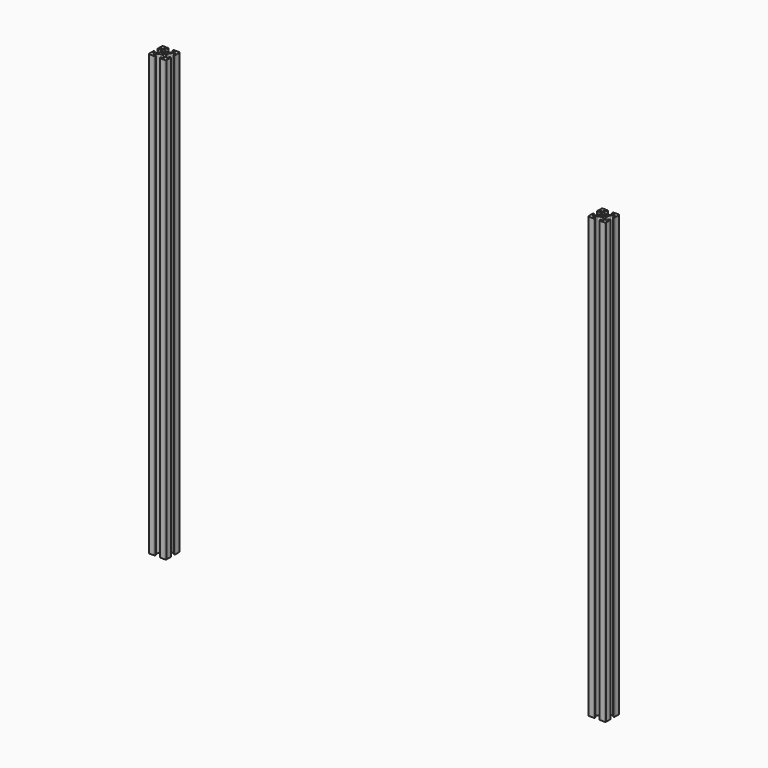
from build123d import *

# Parameters (mm, degrees)
F0_R     = 2.6035
F1_DEPTH = 635
F2_R     = 1.18109
F3_R     = 5.08
F4_R     = 0.762
F5_R     = 1.27


# Not quite as in the source:
# - a fillet or chamfer is up to 0.001 mm smaller than in the source, because OpenCascade refuses the exact size


with BuildPart() as f1:
    # F0 (on Top) → F1 (new body)
    with BuildSketch(Plane.XY):
        Polygon((12.7, 3.2385), (12.7, 12.7), (3.2385, 12.7), (3.2385, 10.3378), (8.7752354349, 10.3378), (2.9459354349, 4.5085), (-2.9459354349, 4.5085), (-8.7752354349, 10.3378), (-3.2385, 10.3378), (-3.2385, 12.7), (-12.7, 12.7), (-12.7, 3.2385), (-10.3378, 3.2385), (-10.3378, 8.7752354349), (-4.5085, 2.9459354349), (-4.5085, -2.9459354349), (-10.3378, -8.7752354349), (-10.3378, -3.2385), (-12.7, -3.2385), (-12.7, -12.7), (-3.2385, -12.7), (-3.2385, -10.3378), (-8.7752354349, -10.3378), (-2.9459354349, -4.5085), (2.9459354349, -4.5085), (8.7752354349, -10.3378), (3.2385, -10.3378), (3.2385, -12.7), (12.7, -12.7), (12.7, -3.2385), (10.3378, -3.2385), (10.3378, -8.7752354349), (4.5085, -2.9459354349), (4.5085, 2.9459354349), (10.3378, 8.7752354349), (10.3378, 3.2385), align=None)
        Circle(F0_R, mode=Mode.SUBTRACT)
    extrude(amount=F1_DEPTH)

    # F2 (radius 1.1811 in the source; OpenCascade refuses exactly that, so slightly less here)
    f2_edges = [f1.edges().sort_by_distance(p)[0] for p in [
        (3.2385, 12.7, 317.5),
        (3.2385, 10.3378, 317.5),
        (-3.2385, 12.7, 317.5),
        (-12.7, 3.2385, 317.5),
        (-3.2385, 10.3378, 317.5),
        (-10.3378, 3.2385, 317.5),
        (12.7, 3.2385, 317.5),
        (10.3378, 3.2385, 317.5),
        (12.7, -3.2385, 317.5),
        (10.3378, -3.2385, 317.5),
        (3.2385, -10.3378, 317.5),
        (-3.2385, -10.3378, 317.5),
        (-10.3378, -3.2385, 317.5),
        (-12.7, -3.2385, 317.5),
        (-3.2385, -12.7, 317.5),
        (3.2385, -12.7, 317.5),
    ]]
    fillet(f2_edges, radius=F2_R)

    # F3
    f3_edges = [f1.edges().sort_by_distance(p)[0] for p in [
        (2.945935, 4.5085, 317.5),
        (-2.945935, 4.5085, 317.5),
        (4.5085, -2.945935, 317.5),
        (4.5085, 2.945935, 317.5),
        (2.945935, -4.5085, 317.5),
        (-2.945935, -4.5085, 317.5),
        (-4.5085, -2.945935, 317.5),
        (-4.5085, 2.945935, 317.5),
    ]]
    fillet(f3_edges, radius=F3_R)

    # F4
    f4_edges = [f1.edges().sort_by_distance(p)[0] for p in [
        (8.775235, 10.3378, 317.5),
        (-8.775235, 10.3378, 317.5),
        (-10.3378, 8.775235, 317.5),
        (-10.3378, -8.775235, 317.5),
        (-8.775235, -10.3378, 317.5),
        (8.775235, -10.3378, 317.5),
        (10.3378, -8.775235, 317.5),
        (10.3378, 8.775235, 317.5),
    ]]
    fillet(f4_edges, radius=F4_R)

    # F5
    f5_edges = [f1.edges().sort_by_distance(p)[0] for p in [
        (-12.7, -12.7, 317.5),
        (12.7, -12.7, 317.5),
        (12.7, 12.7, 317.5),
        (-12.7, 12.7, 317.5),
    ]]
    fillet(f5_edges, radius=F5_R)


with BuildPart() as f6_1:
    # F6: copy of F1
    add(f1.part.moved(Location((635, 0, 0))))


solid = Compound([f1.part, f6_1.part])
